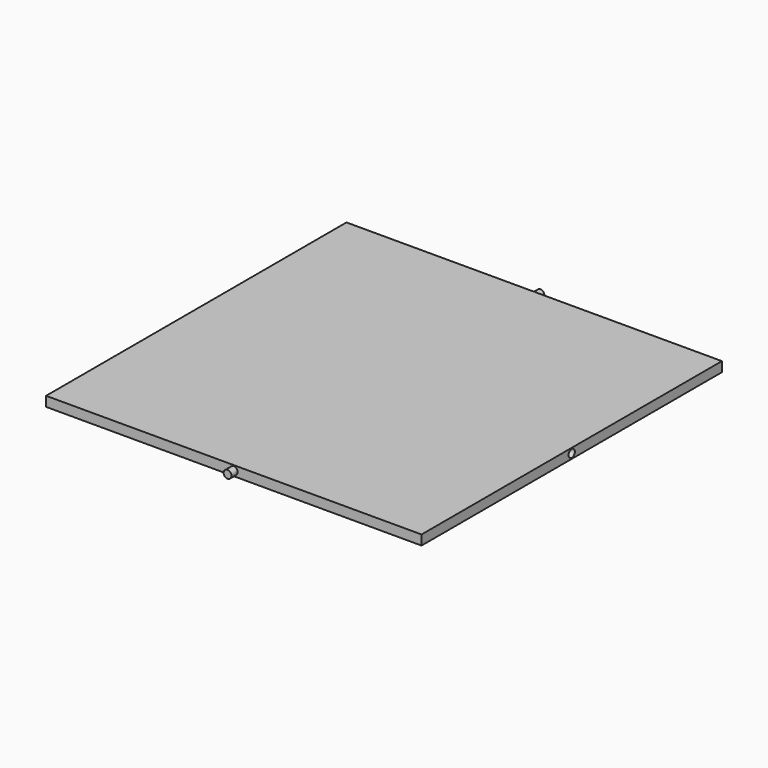
from build123d import *

# Parameters (mm, degrees)
F0_W     = 609.6
F0_H     = 609.6
F1_DEPTH = 7.9375
F2_R     = 6.35
F3_DEPTH = 12.7
F4_R     = 6.35
F5_DEPTH = 12.7
F6_R     = 6.35
F7_DEPTH = 12.7
F8_R     = 6.35
F9_DEPTH = 12.7


# Not quite as in the source:
# - a length typed as a fraction of an inch, garbled in the dataset ("3 / 203.2 mm" for 3/8 in), is restored


with BuildPart() as f1:
    # F0 (on Top) → F1 (new body, symmetric)
    with BuildSketch(Plane.XY):
        Rectangle(F0_W, F0_H)
    extrude(amount=F1_DEPTH, both=True)

    # F2 (on face) → F3 (cut)
    with BuildSketch(Plane.YZ.offset(304.8)):
        Circle(F2_R)
    extrude(amount=-F3_DEPTH, mode=Mode.SUBTRACT)

    # F4 (on face) → F5 (join)
    with BuildSketch(Plane.XZ.offset(304.8)):
        Circle(F4_R)
    extrude(amount=F5_DEPTH)

    # F6 (on face) → F7 (cut)
    with BuildSketch(Plane(origin=(-304.8, 0, 0), x_dir=(0, -1, 0), z_dir=(-1, 0, 0))):
        Circle(F6_R)
    extrude(amount=-F7_DEPTH, mode=Mode.SUBTRACT)

    # F8 (on face) → F9 (join)
    with BuildSketch(Plane(origin=(0, 304.8, 0), x_dir=(-1, 0, 0), z_dir=(0, 1, 0))):
        Circle(F8_R)
    extrude(amount=F9_DEPTH)


solid = f1.part
